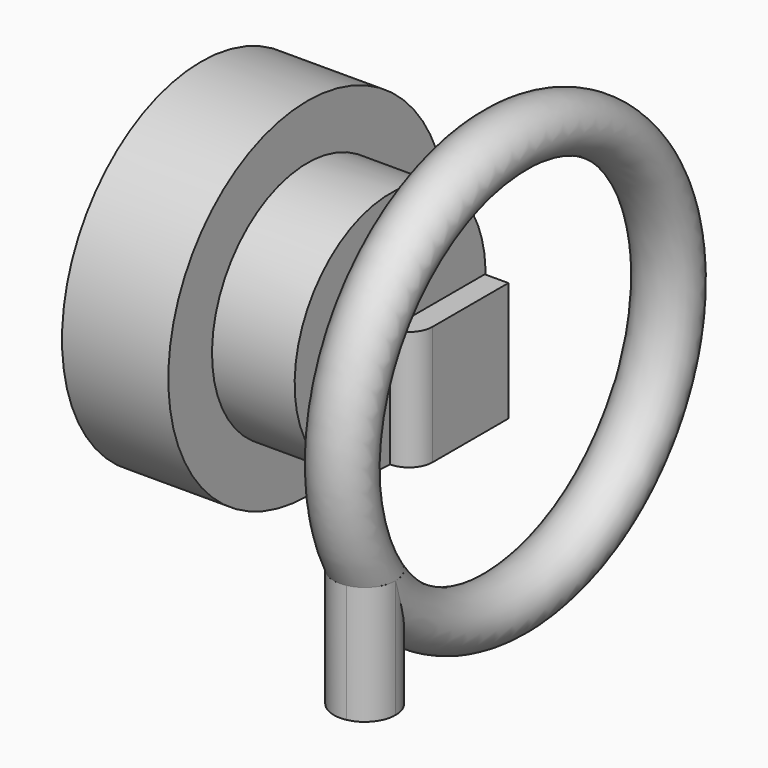
from build123d import *

# Parameters (mm, degrees)
F0_R      = 6.2253326178
F0_W      = 22.8262245655
F0_H      = 11.7288976908
F1_DEPTH  = 25.4
F3_R      = 5.08
F4_DEPTH  = 25.4
F4_FACE_R = 6.625041603
F1_FACE_R = 6.2253326178


with BuildPart() as f1:
    # F0 (on Front) → F1 (new body)
    with BuildSketch(Plane.XZ):
        Polygon((9.2026740313, 47.4568679929), (9.2026740313, 21.8337476254), (32.0288985968, 21.8337476254), (54.8551231623, 21.8337476254), (54.8551231623, 47.4568679929), align=None)
        with Locations((25.803565979, 40.7804250717)):
            Circle(F0_R, mode=Mode.SUBTRACT)
        with Locations((20.615786314, 15.96929878)):
            Rectangle(F0_W, F0_H)
    extrude(amount=F1_DEPTH)

    # F3
    f3_edges = [f1.edges().sort_by_distance(p)[0] for p in [
        (54.855123, -25.4, 34.645308),
    ]]
    fillet(f3_edges, radius=F3_R)


with BuildPart() as f4:
    # F2 (on Top) → F4 (new body)
    with BuildSketch(Plane.XY):
        with BuildLine():
            ThreePointArc((75.7866948843, -56.6520751508), (67.8985414516, -63.1555914879), (75.7866948843, -69.659107825))
            Line((75.7866948843, -69.659107825), (75.7866948843, -56.6520751508))
        make_face()
        with BuildLine():
            Line((75.7866948843, -56.6520751508), (75.7866948843, -69.659107825))
            ThreePointArc((75.7866948843, -69.659107825), (79.6353021716, -67.3700314163), (81.1486246575, -63.1555914879))
            ThreePointArc((81.1486246575, -63.1555914879), (79.6353021716, -58.9411515595), (75.7866948843, -56.6520751508))
        make_face()
    extrude(amount=F4_DEPTH)


with BuildPart() as f5:
    # F4_face (on face) + F1_face (on face) → F5 (revolve)
    with BuildSketch(Plane(origin=(74.5235830545, -63.1555914879, 25.4), x_dir=(1, 0, 0), z_dir=(0, 0, 1))):
        Circle(F4_FACE_R)
    with BuildSketch(Plane(origin=(27.8636251422, -25.4, 29.7978212865), x_dir=(1, 0, 0), z_dir=(0, -1, 0))):
        Polygon((4.1652734545, -7.9640736611), (21.91149802, -7.9640736611), (21.91149802, 17.6590467064), (-18.660951111, 17.6590467064), (-18.660951111, -19.6929713519), (4.1652734545, -19.6929713519), align=None)
        with Locations((-2.0600591632, 10.9826037853)):
            Circle(F1_FACE_R, mode=Mode.SUBTRACT)
    revolve(axis=Axis((29.4888985968, -25.4, 47.4568679929), (1, 0, 0)))


solid = Compound([f1.part, f4.part, f5.part])
